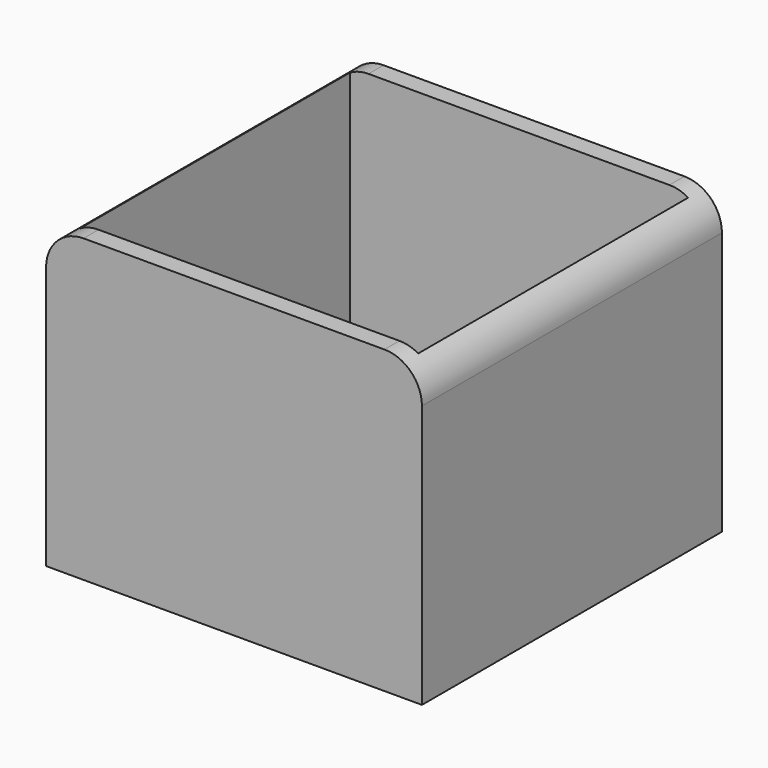
from build123d import *

# Parameters (mm, degrees)
F0_W        = 50.1185376197
F0_H        = 40.0948291644
F1_DEPTH    = 50
F2_T        = -2.5
F3_T1_DEPTH = 75
F4_T1_DEPTH = 75


# Not quite as in the source:
# - a fillet or chamfer that OpenCascade refuses, or shapes differently, is made with other operations: its cross-section is extruded or revolved along the edge and cut away or added


with BuildPart() as f1:
    # F0 (on Front) → F1 (new body)
    with BuildSketch(Plane.XZ):
        with Locations((-0.201604329, 6.9467336871)):
            Rectangle(F0_W, F0_H)
    extrude(amount=F1_DEPTH)

    # F2
    f2_openings = [f1.faces().sort_by_distance(p)[0] for p in [
        (-0.201604, -25, 26.994148),
    ]]
    offset(amount=F2_T, openings=f2_openings)

    # F3: fillet of radius 5 on 1 edges, made by hand

    # F3_s2 → F3_t1 (cut)
    with BuildSketch(Plane.XZ.offset(-12.5)):
        with BuildLine():
            ThreePointArc((24.8576644808, 21.9941482693), (23.3931983867, 25.5296821752), (19.8576644808, 26.9941482693))
            Line((19.8576644808, 26.9941482693), (24.8576644808, 26.9941482693))
            Line((24.8576644808, 26.9941482693), (24.8576644808, 21.9941482693))
        make_face()
    extrude(amount=F3_T1_DEPTH, mode=Mode.SUBTRACT)

    # F4: fillet of radius 5 on 1 edges, made by hand

    # F4_s2 → F4_t1 (cut)
    with BuildSketch(Plane.XZ.offset(-12.5)):
        with BuildLine():
            ThreePointArc((-25.2608731389, 21.9941482693), (-23.7964070448, 25.5296821752), (-20.2608731389, 26.9941482693))
            Line((-20.2608731389, 26.9941482693), (-25.2608731389, 26.9941482693))
            Line((-25.2608731389, 26.9941482693), (-25.2608731389, 21.9941482693))
        make_face()
    extrude(amount=F4_T1_DEPTH, mode=Mode.SUBTRACT)


solid = f1.part
